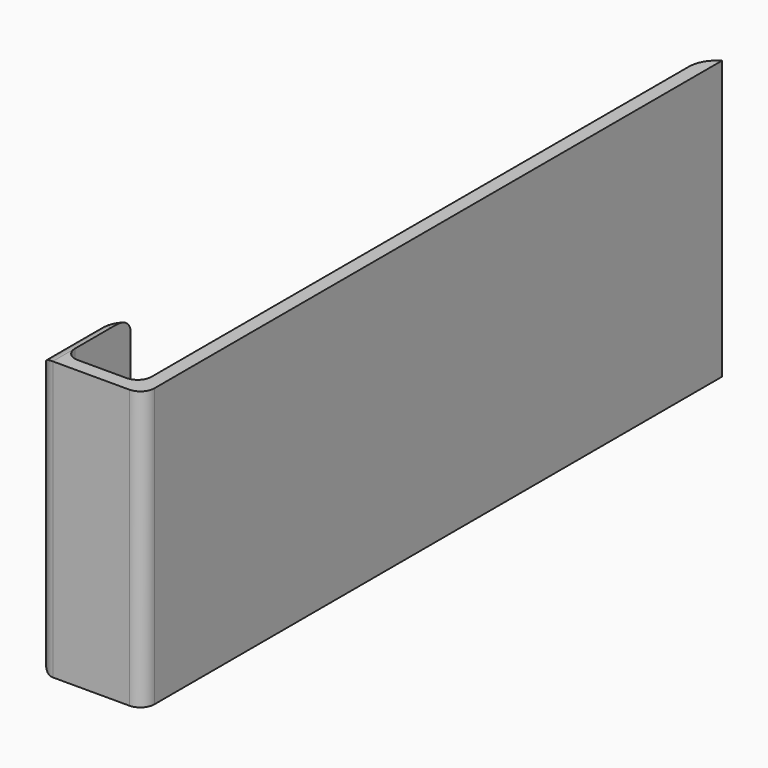
from build123d import *

# Parameters (mm, degrees)
F2_DEPTH    = 19.05
F3_T1_DEPTH = 28.6602540378
F4_R        = 0.9999


# Not quite as in the source:
# - a fillet or chamfer that OpenCascade refuses, or shapes differently, is made with other operations: its cross-section is extruded or revolved along the edge and cut away or added
# - a fillet or chamfer is up to 0.001 mm smaller than in the source, because OpenCascade refuses the exact size
# - a pattern or mirror of a feature is missing from the dataset's text; its kind, count and spacing are read off the source's solid


with BuildPart() as f2:
    # F1 (on Top) → F2 (new body)
    with BuildSketch(Plane.XY):
        Polygon((-7.5, 0), (0, 0), (0, 52), (-1, 52), (-1, 1), (-6.5, 1), (-6.5, 7), (-7.5, 7), align=None)
    extrude(amount=F2_DEPTH)

    # F2_copies: F2 across plane


with BuildPart() as f2_1:
    add(f2.part)
    add(f2.part.mirror(Plane.XY.offset(10)))

    # F3: fillet of radius 2 on 2 edges, made by hand

    # F3_s2 → F3_t1 (cut)
    with BuildSketch(Plane.XY.offset(-4.3301270189)):
        with BuildLine():
            ThreePointArc((-6.5, 7), (-7.2320508076, 6.2679491924), (-7.5, 5.2679491924))
            Line((-7.5, 5.2679491924), (-7.5, 7))
            Line((-7.5, 7), (-6.5, 7))
        make_face()
        with BuildLine():
            ThreePointArc((0, 52), (-0.7320508076, 51.2679491924), (-1, 50.2679491924))
            Line((-1, 50.2679491924), (-1, 52))
            Line((-1, 52), (0, 52))
        make_face()
    extrude(amount=F3_T1_DEPTH, mode=Mode.SUBTRACT)

    # F4 (radius 1 in the source; OpenCascade refuses exactly that, so slightly less here)
    f4_edges = [f2_1.edges().sort_by_distance(p)[0] for p in [
        (-7.5, 2.633975, 0),
        (-7.5, 0, 10),
        (0, 0, 10),
        (-6.5, 1, 10),
        (-1, 1, 10),
        (-7.232051, 6.267949, 0),
        (-7.5, 2.633975, 20),
        (-7.232051, 6.267949, 20),
    ]]
    fillet(f4_edges, radius=F4_R)


solid = f2_1.part
